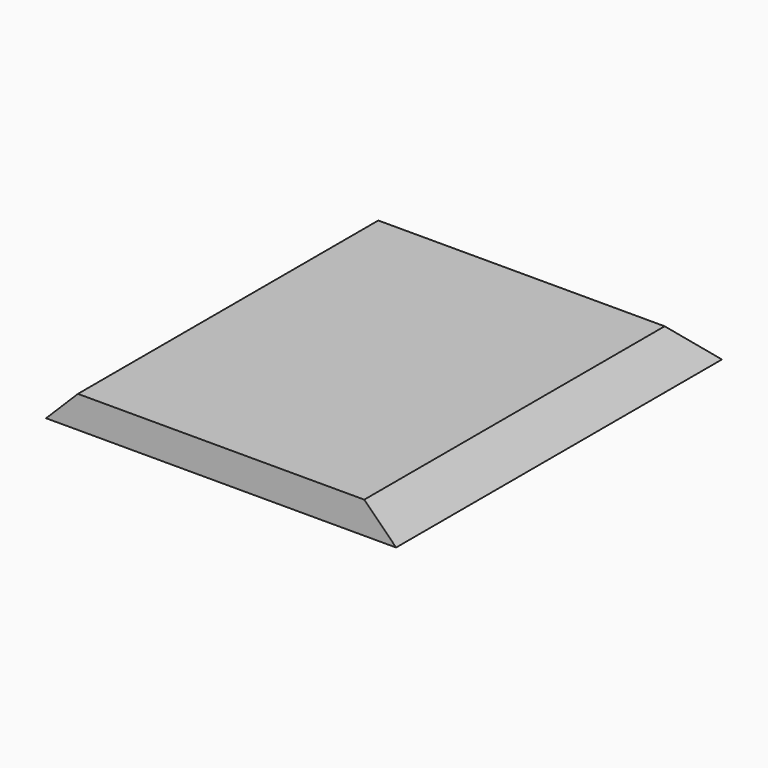
from build123d import *

# Parameters (mm, degrees)
F0_W     = 55
F0_H     = 64
F1_DEPTH = 5
F2_SIZE  = 4.99999


# Not quite as in the source:
# - a fillet or chamfer is up to 0.001 mm smaller than in the source, because OpenCascade refuses the exact size


with BuildPart() as f1:
    # F0 (on Top) → F1 (new body)
    with BuildSketch(Plane.XY):
        with Locations((0, 20.5)):
            Rectangle(F0_W, F0_H)
    extrude(amount=F1_DEPTH)

    # F2 (size 5 in the source; OpenCascade refuses exactly that, so slightly less here)
    f2_edges = [f1.edges().sort_by_distance(p)[0] for p in [
        (-27.5, 20.5, 5),
        (0, 52.5, 5),
        (27.5, 20.5, 5),
    ]]
    chamfer(f2_edges, length=F2_SIZE)


solid = f1.part
